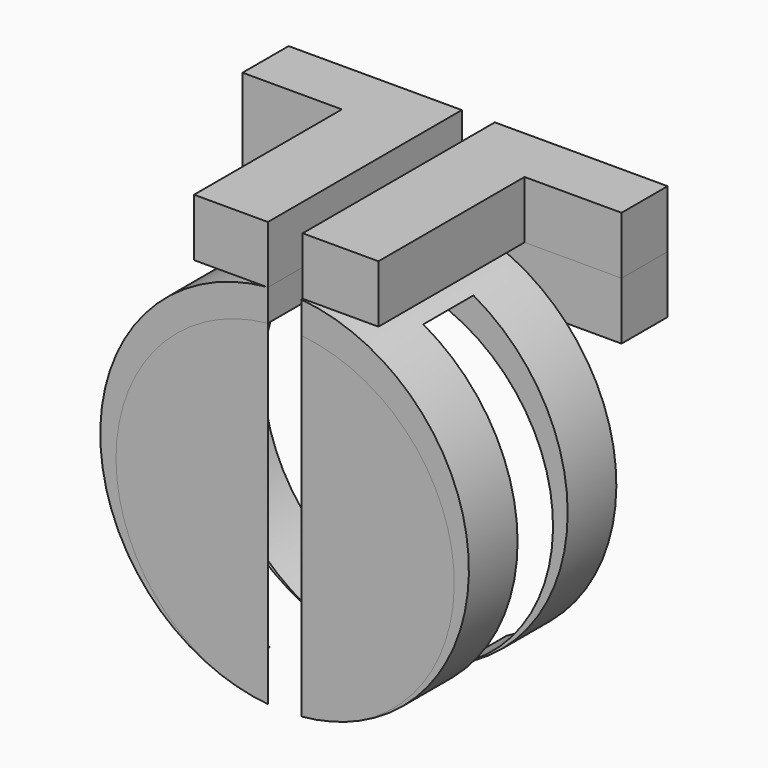
from build123d import *

# Parameters (mm, degrees)
F0_R            = 25.4
F1_DEPTH        = 12.7
F2_W            = 8.63417238
F2_H            = 111.093018204
F3_DEPTH        = 38.1
F5_DEPTH        = 38.1
F6_W            = 4.6048974618
F6_H            = 114.5466864109
F7_DEPTH        = 38.1
F8_DEPTH        = 1.5875
F9_DEPTH        = 76.2
F10_DEPTH       = 25.4
F11_T1_DEPTH    = 64.6536648527
F11_S1_T1_DEPTH = 64.6684980489
F12_W           = 23.8125
F12_H           = 7.9375
F13_DEPTH       = 7.9375
F14_W           = 23.8125
F14_H           = 7.9375
F15_DEPTH       = 7.9375
F16_W           = 10.1776355878
F16_H           = 25.4661563456
F17_DEPTH       = 7.9375
F20_W           = 10.445
F20_H           = 25.1640297145
F21_DEPTH       = 7.938


# Not quite as in the source:
# - a fillet or chamfer that OpenCascade refuses, or shapes differently, is made with other operations: its cross-section is extruded or revolved along the edge and cut away or added


with BuildPart() as f1:
    # F0 (on Front) → F1 (new body, symmetric)
    with BuildSketch(Plane.XZ):
        Circle(F0_R)
    extrude(amount=F1_DEPTH, both=True)

    # F2 (on Right) → F3 (cut, symmetric)
    with BuildSketch(Plane.YZ):
        with Locations((0, -33.3854667842)):
            Rectangle(F2_W, F2_H)
    extrude(amount=F3_DEPTH, both=True, mode=Mode.SUBTRACT)

    # F4 (on face) → F5 (cut, symmetric)
    with BuildSketch(Plane.XZ.offset(12.7)):
        with BuildLine():
            ThreePointArc((-8.7293650817, -23.8528443853), (0.834589374, -25.3862848912), (10.2771759058, -23.2279929267))
            ThreePointArc((10.2771759058, -23.2279929267), (-0.6911145239, 21.0221106841), (-8.7293650817, -23.8528443853))
        make_face()
    extrude(amount=F5_DEPTH, both=True, mode=Mode.SUBTRACT)

    # F6 (on Top) → F7 (cut, symmetric)
    with BuildSketch(Plane.XY):
        with Locations((0, -20.7220129669)):
            Rectangle(F6_W, F6_H)
    extrude(amount=F7_DEPTH, both=True, mode=Mode.SUBTRACT)

    # F12 (on face) → F13 (join)
    with BuildSketch(Plane(origin=(0, 12.7, 0), x_dir=(-1, 0, 0), z_dir=(0, 1, 0))):
        with Locations((-14.2086987309, 21.3266790306)):
            Rectangle(F12_W, F12_H)
    extrude(amount=F13_DEPTH)

    # F14 (on face) → F15 (join)
    with BuildSketch(Plane(origin=(0, 12.7, 0), x_dir=(-1, 0, 0), z_dir=(0, 1, 0))):
        with Locations((14.2086987309, 21.3266790306)):
            Rectangle(F14_W, F14_H)
        Polygon((2.2461330518, 25.2954290306), (2.3024487309, 25.2954290306), (26.1149487309, 25.2954290306), (26.1149487309, 33.2456290306), (2.2461330518, 33.2456290306), align=None)
    extrude(amount=F15_DEPTH)

    # F16 (on face) → F17 (join)
    with BuildSketch(Plane.XY.offset(33.2456290306)):
        with Locations((-7.3349508457, -0.0330781728)):
            Rectangle(F16_W, F16_H)
    extrude(amount=-F17_DEPTH)


with BuildPart() as f8:
    # F4 (on face) → F8 (new body)
    with BuildSketch(Plane.XZ.offset(12.7)):
        with BuildLine():
            ThreePointArc((-8.7293650817, -23.8528443853), (0.834589374, -25.3862848912), (10.2771759058, -23.2279929267))
            ThreePointArc((10.2771759058, -23.2279929267), (-0.6911145239, 21.0221106841), (-8.7293650817, -23.8528443853))
        make_face()
    extrude(amount=-F8_DEPTH)

    # F6 (on Top) → F9 (cut)
    with BuildSketch(Plane.XY):
        with Locations((0, -20.7220129669)):
            Rectangle(F6_W, F6_H)
    extrude(amount=-F9_DEPTH, mode=Mode.SUBTRACT)

    # F6 (on Top) → F10 (cut, symmetric)
    with BuildSketch(Plane.XY):
        with Locations((0, -20.7220129669)):
            Rectangle(F6_W, F6_H)
    extrude(amount=F10_DEPTH, both=True, mode=Mode.SUBTRACT)

    # F11: fillet of radius 5.08 on 1 edges, made by hand

    # F11_s2 → F11_t1 (cut)
    with BuildSketch(Plane.XY.offset(-34.5179706237)):
        with BuildLine():
            ThreePointArc((-5.9914653682, -11.1125), (-3.983419054, -11.52622204), (-2.3024487309, -12.7))
            Line((-2.3024487309, -12.7), (-2.3024487309, -11.1125))
            Line((-2.3024487309, -11.1125), (-5.9914653682, -11.1125))
        make_face()
    extrude(amount=F11_T1_DEPTH, mode=Mode.SUBTRACT)

    # F11#s1: fillet of radius 5.08 on 1 edges, made by hand

    # F11_s1_s2 → F11_s1_t1 (cut)
    with BuildSketch(Plane.XY.offset(-34.5179706237)):
        with BuildLine():
            ThreePointArc((2.3024487309, -12.7), (3.983419054, -11.52622204), (5.9914653682, -11.1125))
            Line((5.9914653682, -11.1125), (2.3024487309, -11.1125))
            Line((2.3024487309, -11.1125), (2.3024487309, -12.7))
        make_face()
    extrude(amount=F11_S1_T1_DEPTH, mode=Mode.SUBTRACT)


with BuildPart() as f21:
    # F20 (on face) → F21 (new body)
    with BuildSketch(Plane.XY.offset(25.2954290306)):
        Polygon((26.1149487309, 20.6375), (2.3024487309, 20.6375), (2.3024487309, 12.7), (12.7474487309, 12.7), (26.1149487309, 12.7), align=None)
        with Locations((7.5249487309, 0.1179851428)):
            Rectangle(F20_W, F20_H)
    extrude(amount=F21_DEPTH)


solid = Compound([f1.part, f8.part, f21.part])
